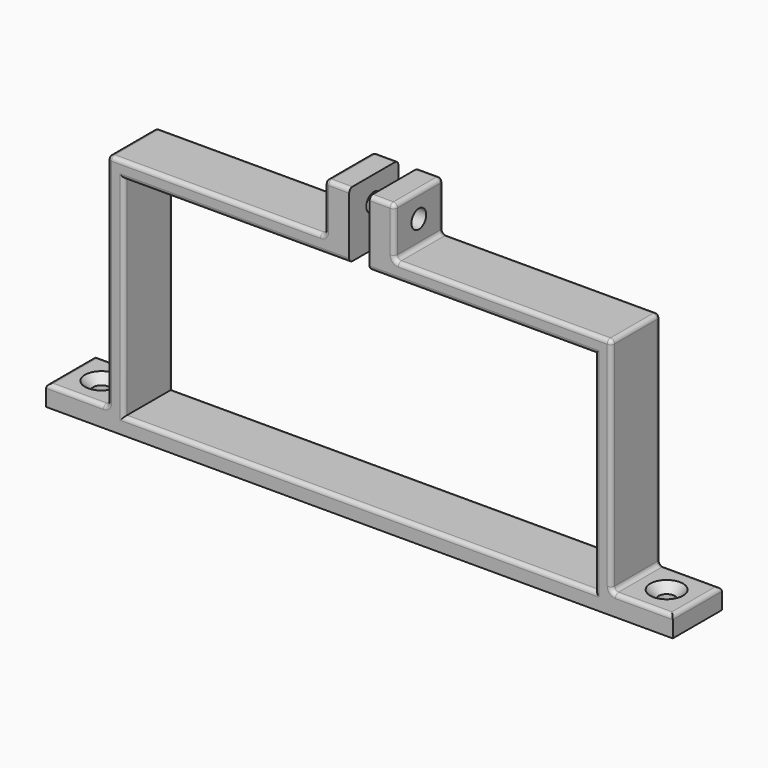
from build123d import *

# Parameters (mm, degrees)
F1_DEPTH = 15
F2_R     = 2.25
F3_DEPTH = 25
F5_R     = 2.25
F6_DEPTH = 1.5
F7_W     = 15
F7_H     = 15
F7_R     = 2
F8_DEPTH = 5
F9_R     = 1
F10_SIZE = 2


with BuildPart() as f1:
    # F0 (on Front) → F1 (new body)
    with BuildSketch(Plane.XZ):
        Polygon((-57.5, -25.5), (-57.5, 25.5), (-8.5, 25.5), (-2.5, 25.5), (-2.5, 41.5), (-8.5, 41.5), (-8.5, 29.5), (-61.5, 29.5), (-61.5, -29.5), (61.5, -29.5), (61.5, 29.5), (8.5, 29.5), (8.5, 41.5), (2.5, 41.5), (2.5, 25.5), (8.5, 25.5), (57.5, 25.5), (57.5, -25.5), align=None)
    extrude(amount=F1_DEPTH)

    # F2 (on face) → F3 (cut)
    with BuildSketch(Plane.YZ.offset(8.5)):
        with Locations((-7.5, 35.5)):
            Circle(F2_R)
    extrude(amount=-F3_DEPTH, mode=Mode.SUBTRACT)

    # F5 (on face) → F6 (cut)
    with BuildSketch(Plane(origin=(-8.5, 0, 0), x_dir=(0, -1, 0), z_dir=(-1, 0, 0))):
        Polygon((9.45799692, 31.9645252943), (11.5408093696, 35.4279377204), (9.5828124496, 38.9634124261), (5.54200308, 39.0354747057), (3.4591906304, 35.5720622796), (5.4171875504, 32.0365875739), align=None)
        with Locations((7.5, 35.5)):
            Circle(F5_R, mode=Mode.SUBTRACT)
    extrude(amount=-F6_DEPTH, mode=Mode.SUBTRACT)

    # F7 (on face) → F8 (join)
    with BuildSketch(Plane(origin=(0, 0, -29.5), x_dir=(1, 0, 0), z_dir=(0, 0, -1))):
        with Locations((-69, 7.5)):
            Rectangle(F7_W, F7_H)
        with Locations((-69, 7.5)):
            Circle(F7_R, mode=Mode.SUBTRACT)
        with Locations((69, 7.5)):
            Rectangle(F7_W, F7_H)
        with Locations((69, 7.5)):
            Circle(F7_R, mode=Mode.SUBTRACT)
    extrude(amount=-F8_DEPTH)

    # F9
    f9_edges = [f1.edges().sort_by_distance(p)[0] for p in [
        (30, 0, 25.5),
        (57.5, 0, 0),
        (-30, 0, 25.5),
        (-57.5, 0, 0),
        (0, 0, -25.5),
        (-30, -15, 25.5),
        (30, -15, 25.5),
        (-57.5, -15, 0),
        (0, -15, -25.5),
        (57.5, -15, 0),
        (-69, -15, -24.5),
        (-76.5, -7.5, -24.5),
        (-69, 0, -24.5),
        (69, 0, -24.5),
        (76.5, -7.5, -24.5),
        (69, -15, -24.5),
        (61.5, -7.5, -24.5),
        (-61.5, -7.5, -24.5),
        (-35, -15, 29.5),
        (-35, 0, 29.5),
        (35, 0, 29.5),
        (8.5, -7.5, 29.5),
        (-8.5, -7.5, 29.5),
        (-8.5, -4.500597, 37.303768),
        (-8.5, -15, 35.5),
        (-8.5, 0, 35.5),
        (-8.5, -7.5, 41.5),
        (8.5, -7.5, 41.5),
        (8.5, -15, 35.5),
        (35, -15, 29.5),
        (61.5, -7.5, 29.5),
        (-61.5, -7.5, 29.5),
        (5.5, 0, 41.5),
        (-5.5, 0, 41.5),
        (-5.5, -15, 41.5),
        (5.5, -15, 41.5),
        (-61.5, -15, 2.5),
        (61.5, -15, 2.5),
        (8.5, 0, 35.5),
        (61.5, 0, 2.5),
        (-61.5, 0, 2.5),
    ]]
    fillet(f9_edges, radius=F9_R)

    # F10
    f10_edges = [f1.edges().sort_by_distance(p)[0] for p in [
        (67, -7.5, -24.5),
        (-71, -7.5, -24.5),
    ]]
    chamfer(f10_edges, length=F10_SIZE)


solid = f1.part
